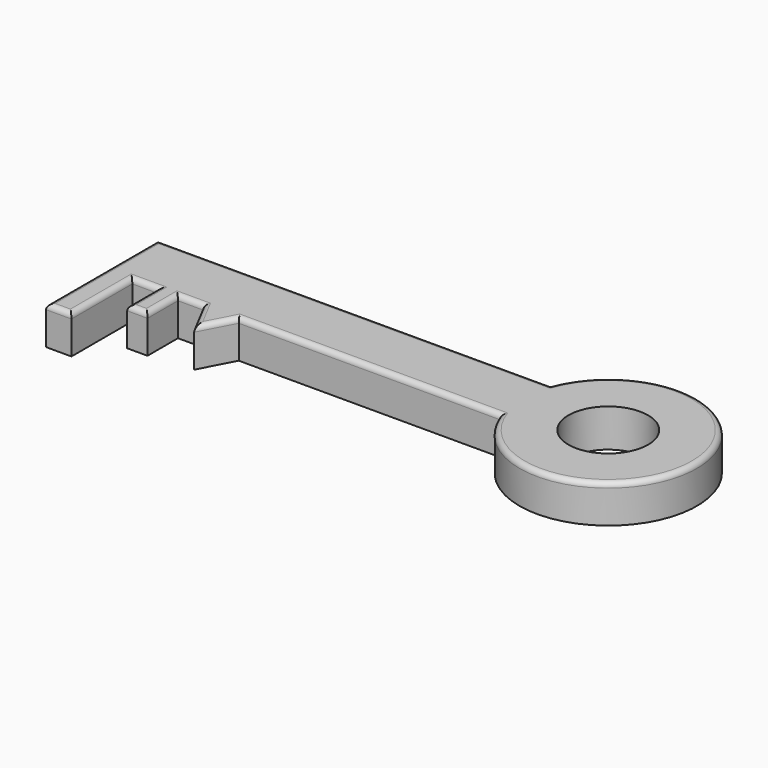
from build123d import *

# Parameters (mm, degrees)
F0_W     = 10
F0_H     = 30
F0_W_2   = 8
F0_H_2   = 15
F0_R     = 15.7140180489
F1_DEPTH = 15
F2_R     = 2


with BuildPart() as f1:
    # F0 (on Top) → F1 (new body)
    with BuildSketch(Plane.XY):
        Polygon((72.5661343038, 22.2410344053), (-82.4338656962, 22.2410344053), (-82.4338656962, -2.7589655947), (-72.4338656962, -2.7589655947), (-62.4338656962, -2.7589655947), (-54.4338656962, -2.7589655947), (-44.4338656962, -2.7589655947), (-30.4338656962, -2.7589655947), (72.5661343038, -2.7589655947), align=None)
        with Locations((-77.4338656962, -17.7589655947)):
            Rectangle(F0_W, F0_H)
        with Locations((-58.4338656962, -10.2589655947)):
            Rectangle(F0_W_2, F0_H_2)
        Polygon((-37.4338656962, -16.0254647561), (-30.4338656962, -2.7589655947), (-44.4338656962, -2.7589655947), align=None)
        with BuildLine():
            ThreePointArc((72.5661343038, -2.7589655947), (140.2578763804, 9.7410344053), (72.5661343038, 22.2410344053))
            Line((72.5661343038, 22.2410344053), (72.5661343038, -2.7589655947))
        make_face()
        with Locations((105.2578763804, 9.7410344053)):
            Circle(F0_R, mode=Mode.SUBTRACT)
    extrude(amount=F1_DEPTH)

    # F2
    f2_edges = [f1.edges().sort_by_distance(p)[0] for p in [
        (-82.433866, -5.258966, 15),
        (-4.933866, 22.241034, 15),
        (-72.433866, -17.758966, 15),
        (-77.433866, -32.758966, 15),
        (-67.433866, -2.758966, 15),
        (-62.433866, -10.258966, 15),
        (-58.433866, -17.758966, 15),
        (-54.433866, -10.258966, 15),
        (-40.933866, -9.392215, 15),
        (21.066134, -2.758966, 15),
        (-33.933866, -9.392215, 15),
        (140.257876, 9.741034, 15),
        (-49.433866, -2.758966, 15),
    ]]
    fillet(f2_edges, radius=F2_R)


solid = f1.part
